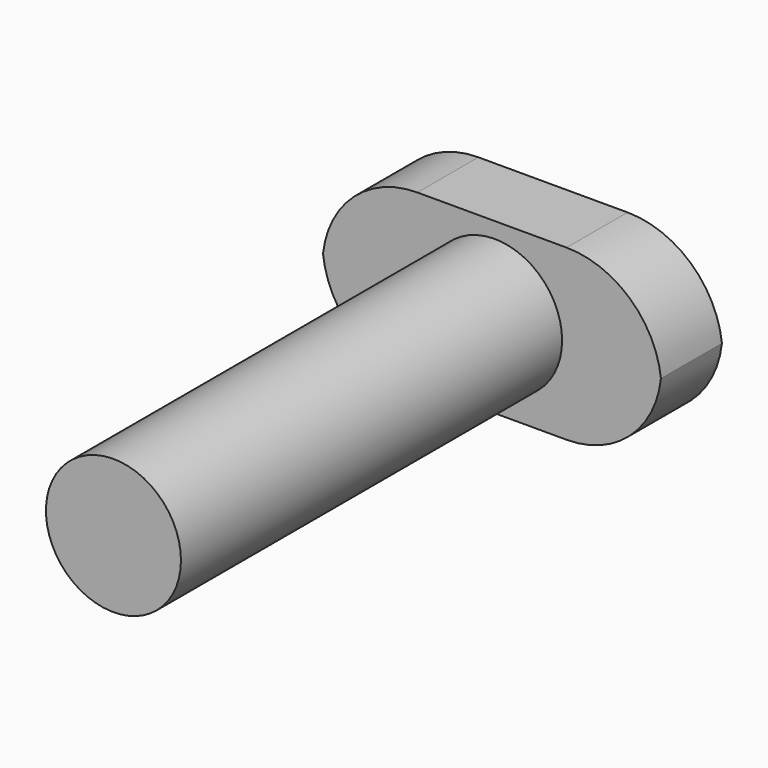
from build123d import *

# Parameters (mm, degrees)
F0_R          = 7.380765
F1_DEPTH      = 57.7
F2_W          = 37.0757319033
F2_H          = 8.3348543849
F3_DEPTH      = 9.1
F3_DEPTH_BACK = 9.4
F4_T1_DEPTH   = 60.2404459759


# Not quite as in the source:
# - a fillet or chamfer that OpenCascade refuses, or shapes differently, is made with other operations: its cross-section is extruded or revolved along the edge and cut away or added


with BuildPart() as f1:
    # F0 (on Front) → F1 (new body)
    with BuildSketch(Plane.XZ):
        Circle(F0_R)
    extrude(amount=F1_DEPTH)

    # F2 (on Top) → F3 (join, two sides)
    with BuildSketch(Plane.XY) as f3_sk:
        with Locations((-0.2874098718, -1.4370438876)):
            Rectangle(F2_W, F2_H)
    extrude(amount=F3_DEPTH)
    extrude(f3_sk.sketch, amount=-F3_DEPTH_BACK)

    # F4: fillet of radius 10.3811183182 on 4 edges, made by hand

    # F4_s2 → F4_t1 (cut)
    with BuildSketch(Plane.XZ.offset(-28.6831791004)):
        with BuildLine():
            ThreePointArc((-18.8252758235, 0.9811183182), (-15.7847166644, -6.3594408409), (-8.4441575053, -9.4))
            Line((-8.4441575053, -9.4), (-18.8252758235, -9.4))
            Line((-18.8252758235, -9.4), (-18.8252758235, 0.9811183182))
        make_face()
        with BuildLine():
            ThreePointArc((-8.4441575053, 9.1), (-15.7847166644, 6.0594408409), (-18.8252758235, -1.2811183182))
            Line((-18.8252758235, -1.2811183182), (-18.8252758235, 9.1))
            Line((-18.8252758235, 9.1), (-8.4441575053, 9.1))
        make_face()
        with BuildLine():
            ThreePointArc((7.8693377616, 9.1), (15.2098969207, 6.0594408409), (18.2504560798, -1.2811183182))
            Line((18.2504560798, -1.2811183182), (18.2504560798, 9.1))
            Line((18.2504560798, 9.1), (7.8693377616, 9.1))
        make_face()
        with BuildLine():
            ThreePointArc((18.2504560798, 0.9811183182), (15.2098969207, -6.3594408409), (7.8693377616, -9.4))
            Line((7.8693377616, -9.4), (18.2504560798, -9.4))
            Line((18.2504560798, -9.4), (18.2504560798, 0.9811183182))
        make_face()
    extrude(amount=F4_T1_DEPTH, mode=Mode.SUBTRACT)


solid = f1.part
